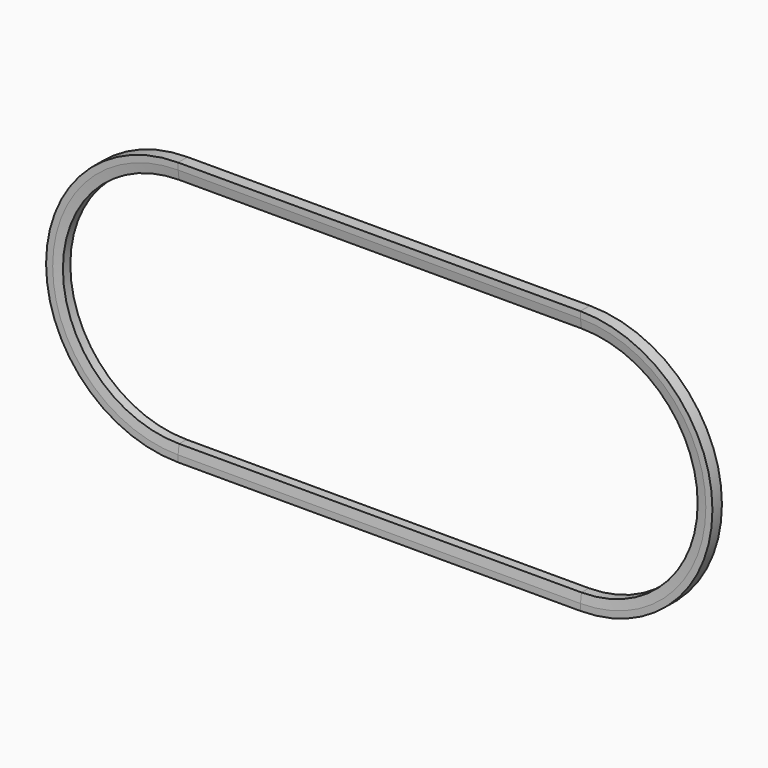
from build123d import *


with BuildPart() as f2:
    # F2: sweep along a path in F1
    with BuildLine(Plane.XZ) as f2_path:
        Line((0, 266.9991701841), (865.7673536606, 266.9991701841))
        ThreePointArc((865.7673536606, 266.9991701841), (1132.7665238447, 0), (865.7673536606, -266.9991701841))
        Line((865.7673536606, -266.9991701841), (0, -266.9991701841))
        ThreePointArc((0, -266.9991701841), (-266.9991701841, 0), (0, 266.9991701841))
    # F0 (on Right) → F2 (sweep)
    with BuildSketch(Plane.YZ):
        Polygon((10.0134903274, 250.0092067223), (12.7307107569, 269.8237648334), (12.7307107569, 283.9983403683), (-12.7660859497, 283.9749474953), (-12.7400761126, 269.800395824), (-9.9865012549, 249.9908570736), align=None)
    sweep(path=f2_path.line)


solid = f2.part
